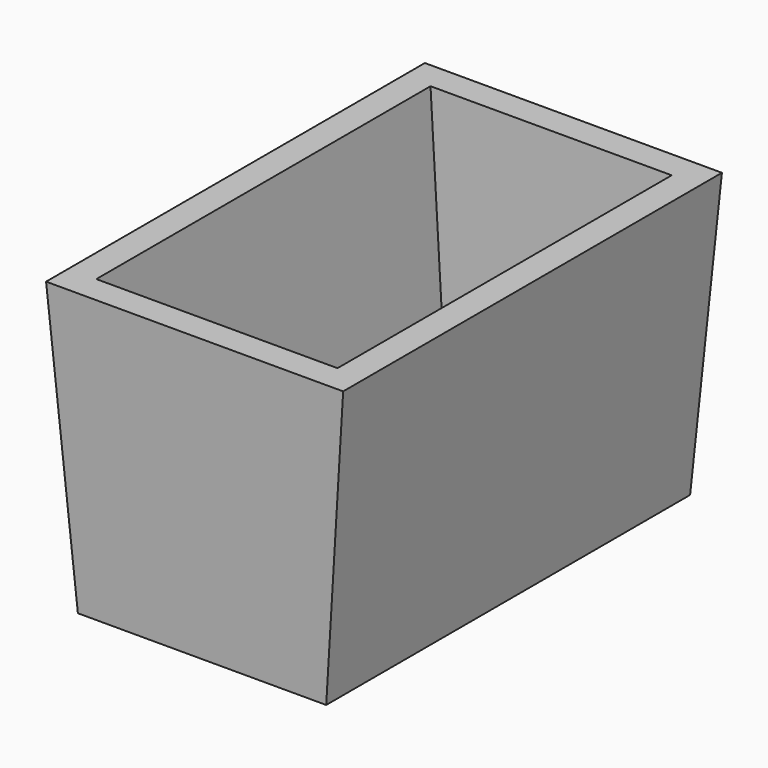
from build123d import *

# Parameters (mm, degrees)
F2_W = 406.4
F2_H = 647.7
F1_W = 339.725
F1_H = 622.3
F4_T = -38.1


with BuildPart() as f3:
    # F2 (on offset) → F3 section 0
    with BuildSketch(Plane.XY.offset(393.7)):
        Rectangle(F2_W, F2_H)
    # F1 (on Top) → F3 section 1
    with BuildSketch(Plane.XY):
        Rectangle(F1_W, F1_H)
    loft()

    # F4
    f4_openings = [f3.faces().sort_by_distance(p)[0] for p in [
        (0, 0, 393.7),
    ]]
    offset(amount=F4_T, openings=f4_openings)


solid = f3.part
